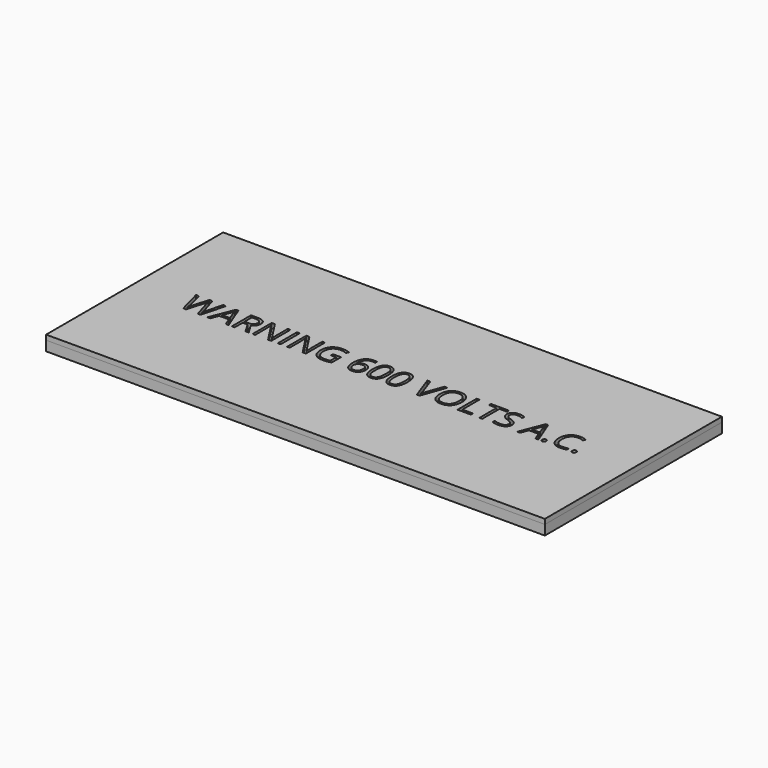
from build123d import *

# Parameters (mm, degrees)
F0_W         = 101.6
F0_H         = 45.08
F1_DEPTH     = 2
F2_DEPTH     = 1
F3_TEXT_SIZE = 6.8183776585
F4_DEPTH     = 1


# Not quite as in the source:
# - Text() gives the source's letters only with a copy of the font that has no kerning and outlines rounded to 1/6400 em; it was checked with that copy


with BuildPart() as f1:
    # F0 (on Top) → F1 (new body)
    with BuildSketch(Plane.XY):
        with Locations((13.6351218998, -1.0988798803)):
            Rectangle(F0_W, F0_H)
    extrude(amount=F1_DEPTH)


with BuildPart() as f2:
    # F2 (new): a face of the model
    f2_faces = [f1.part.faces().sort_by_distance(p)[0] for p in [
        (13.6351218998, -1.0988798803, 2),
    ]]
    extrude(f2_faces, amount=F2_DEPTH)

    # F3 (on face) → F4 (cut)
    with BuildSketch(Plane.XY.offset(3)):
        with Locations((-27.1648781002, -2.9487813031)):
            Text('WARNING 600 VOLTS A.C.', F3_TEXT_SIZE, font='Open Sans', text_align=(TextAlign.LEFT, TextAlign.BOTTOM))
    extrude(amount=-F4_DEPTH, mode=Mode.SUBTRACT)


solid = Compound([f1.part, f2.part])
